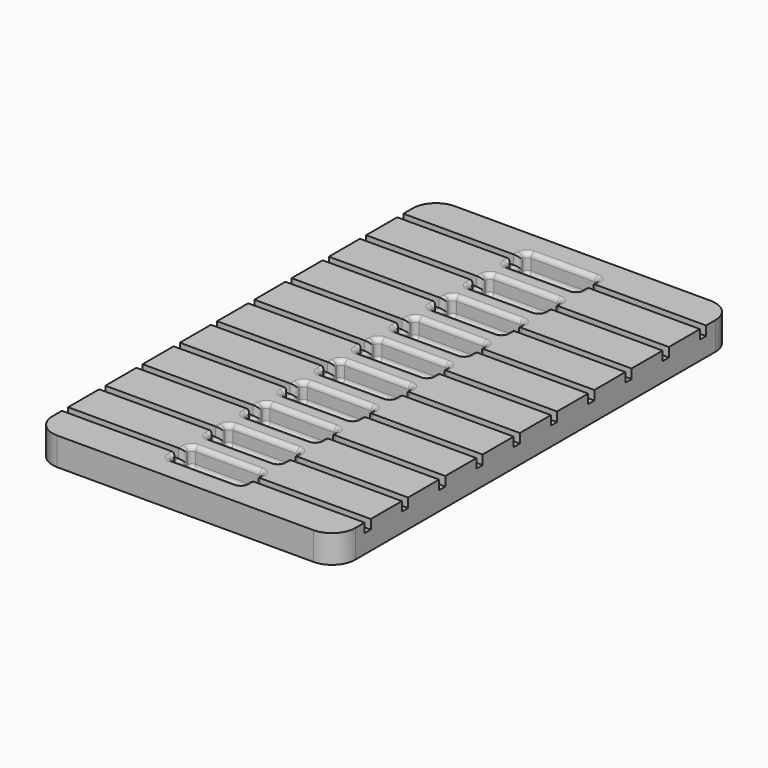
from build123d import *

# Parameters (mm, degrees)
F0_W     = 49.53
F0_H     = 81.28
F1_DEPTH = 4.572
F2_W     = 11.938
F2_H     = 4.572
F3_DEPTH = 3.302
F4_W     = 18.796
F4_H     = 1.27
F5_DEPTH = 1.524
F6_R     = 0.762
F7_R     = 3.81


with BuildPart() as f1:
    # F0 (on Top) → F1 (new body)
    with BuildSketch(Plane.XY):
        with Locations((24.765, 40.64)):
            Rectangle(F0_W, F0_H)
    extrude(amount=F1_DEPTH)

    # F2 (on face) → F3 (cut)
    with BuildSketch(Plane.XY.offset(4.572)):
        with Locations((24.765, 6.35)):
            Rectangle(F2_W, F2_H)
        with Locations((24.765, 13.97)):
            Rectangle(F2_W, F2_H)
        with Locations((24.765, 21.59)):
            Rectangle(F2_W, F2_H)
        with Locations((24.765, 29.21)):
            Rectangle(F2_W, F2_H)
        with Locations((24.765, 36.83)):
            Rectangle(F2_W, F2_H)
        with Locations((24.765, 44.45)):
            Rectangle(F2_W, F2_H)
        with Locations((24.765, 52.07)):
            Rectangle(F2_W, F2_H)
        with Locations((24.765, 59.69)):
            Rectangle(F2_W, F2_H)
        with Locations((24.765, 67.31)):
            Rectangle(F2_W, F2_H)
        with Locations((24.765, 74.93)):
            Rectangle(F2_W, F2_H)
    extrude(amount=-F3_DEPTH, mode=Mode.SUBTRACT)

    # F4 (on face) → F5 (cut)
    with BuildSketch(Plane.XY.offset(4.572)):
        with Locations((40.132, 6.35)):
            Rectangle(F4_W, F4_H)
        with Locations((9.398, 6.35)):
            Rectangle(F4_W, F4_H)
        with Locations((9.398, 13.97)):
            Rectangle(F4_W, F4_H)
        with Locations((40.132, 13.97)):
            Rectangle(F4_W, F4_H)
        with Locations((9.398, 21.59)):
            Rectangle(F4_W, F4_H)
        with Locations((40.132, 21.59)):
            Rectangle(F4_W, F4_H)
        with Locations((9.398, 29.21)):
            Rectangle(F4_W, F4_H)
        with Locations((40.132, 29.21)):
            Rectangle(F4_W, F4_H)
        with Locations((9.398, 36.83)):
            Rectangle(F4_W, F4_H)
        with Locations((40.132, 36.83)):
            Rectangle(F4_W, F4_H)
        with Locations((9.398, 44.45)):
            Rectangle(F4_W, F4_H)
        with Locations((40.132, 44.45)):
            Rectangle(F4_W, F4_H)
        with Locations((9.398, 52.07)):
            Rectangle(F4_W, F4_H)
        with Locations((40.132, 52.07)):
            Rectangle(F4_W, F4_H)
        with Locations((9.398, 59.69)):
            Rectangle(F4_W, F4_H)
        with Locations((40.132, 59.69)):
            Rectangle(F4_W, F4_H)
        with Locations((9.398, 67.31)):
            Rectangle(F4_W, F4_H)
        with Locations((40.132, 67.31)):
            Rectangle(F4_W, F4_H)
        with Locations((9.398, 74.93)):
            Rectangle(F4_W, F4_H)
        with Locations((40.132, 74.93)):
            Rectangle(F4_W, F4_H)
    extrude(amount=-F5_DEPTH, mode=Mode.SUBTRACT)

    # F6
    f6_edges = [f1.edges().sort_by_distance(p)[0] for p in [
        (18.796, 4.064, 2.921),
        (30.734, 4.064, 2.921),
        (24.765, 4.064, 4.572),
        (24.765, 4.064, 1.27),
        (18.796, 7.8105, 4.572),
        (18.796, 6.985, 3.81),
        (18.796, 6.35, 3.048),
        (18.796, 5.715, 3.81),
        (18.796, 4.8895, 4.572),
        (18.796, 6.35, 1.27),
        (18.796, 8.636, 2.921),
        (30.734, 4.8895, 4.572),
        (30.734, 5.715, 3.81),
        (30.734, 6.35, 3.048),
        (30.734, 6.985, 3.81),
        (30.734, 7.8105, 4.572),
        (30.734, 8.636, 2.921),
        (30.734, 6.35, 1.27),
        (24.765, 8.636, 4.572),
        (24.765, 8.636, 1.27),
        (18.796, 15.4305, 4.572),
        (18.796, 14.605, 3.81),
        (18.796, 13.97, 3.048),
        (18.796, 13.335, 3.81),
        (18.796, 12.5095, 4.572),
        (18.796, 11.684, 2.921),
        (18.796, 13.97, 1.27),
        (18.796, 16.256, 2.921),
        (18.796, 23.0505, 4.572),
        (18.796, 22.225, 3.81),
        (18.796, 21.59, 3.048),
        (18.796, 20.955, 3.81),
        (18.796, 20.1295, 4.572),
        (18.796, 19.304, 2.921),
        (18.796, 21.59, 1.27),
        (18.796, 23.876, 2.921),
        (18.796, 30.6705, 4.572),
        (18.796, 29.845, 3.81),
        (18.796, 29.21, 3.048),
        (18.796, 28.575, 3.81),
        (18.796, 27.7495, 4.572),
        (18.796, 26.924, 2.921),
        (18.796, 29.21, 1.27),
        (18.796, 31.496, 2.921),
        (18.796, 38.2905, 4.572),
        (18.796, 37.465, 3.81),
        (18.796, 36.83, 3.048),
        (18.796, 36.195, 3.81),
        (18.796, 35.3695, 4.572),
        (18.796, 34.544, 2.921),
        (18.796, 36.83, 1.27),
        (18.796, 39.116, 2.921),
        (18.796, 45.9105, 4.572),
        (18.796, 45.085, 3.81),
        (18.796, 44.45, 3.048),
        (18.796, 43.815, 3.81),
        (18.796, 42.9895, 4.572),
        (18.796, 42.164, 2.921),
        (18.796, 44.45, 1.27),
        (18.796, 46.736, 2.921),
        (18.796, 53.5305, 4.572),
        (18.796, 52.705, 3.81),
        (18.796, 52.07, 3.048),
        (18.796, 51.435, 3.81),
        (18.796, 50.6095, 4.572),
        (18.796, 49.784, 2.921),
        (18.796, 52.07, 1.27),
        (18.796, 54.356, 2.921),
        (18.796, 61.1505, 4.572),
        (18.796, 60.325, 3.81),
        (18.796, 59.69, 3.048),
        (18.796, 59.055, 3.81),
        (18.796, 58.2295, 4.572),
        (18.796, 57.404, 2.921),
        (18.796, 59.69, 1.27),
        (18.796, 61.976, 2.921),
        (18.796, 68.7705, 4.572),
        (18.796, 67.945, 3.81),
        (18.796, 67.31, 3.048),
        (18.796, 66.675, 3.81),
        (18.796, 65.8495, 4.572),
        (18.796, 65.024, 2.921),
        (18.796, 67.31, 1.27),
        (18.796, 69.596, 2.921),
        (18.796, 76.3905, 4.572),
        (18.796, 75.565, 3.81),
        (18.796, 74.93, 3.048),
        (18.796, 74.295, 3.81),
        (18.796, 73.4695, 4.572),
        (18.796, 72.644, 2.921),
        (18.796, 74.93, 1.27),
        (18.796, 77.216, 2.921),
        (30.734, 73.4695, 4.572),
        (30.734, 74.295, 3.81),
        (30.734, 74.93, 3.048),
        (30.734, 75.565, 3.81),
        (30.734, 76.3905, 4.572),
        (30.734, 77.216, 2.921),
        (30.734, 74.93, 1.27),
        (30.734, 72.644, 2.921),
        (30.734, 65.8495, 4.572),
        (30.734, 66.675, 3.81),
        (30.734, 67.31, 3.048),
        (30.734, 67.945, 3.81),
        (30.734, 68.7705, 4.572),
        (30.734, 69.596, 2.921),
        (30.734, 67.31, 1.27),
        (30.734, 65.024, 2.921),
        (30.734, 58.2295, 4.572),
        (30.734, 59.055, 3.81),
        (30.734, 59.69, 3.048),
        (30.734, 60.325, 3.81),
        (30.734, 61.1505, 4.572),
        (30.734, 61.976, 2.921),
        (30.734, 59.69, 1.27),
        (30.734, 57.404, 2.921),
        (30.734, 50.6095, 4.572),
        (30.734, 51.435, 3.81),
        (30.734, 52.07, 3.048),
        (30.734, 52.705, 3.81),
        (30.734, 53.5305, 4.572),
        (30.734, 54.356, 2.921),
        (30.734, 52.07, 1.27),
        (30.734, 49.784, 2.921),
        (30.734, 42.9895, 4.572),
        (30.734, 43.815, 3.81),
        (30.734, 44.45, 3.048),
        (30.734, 45.085, 3.81),
        (30.734, 45.9105, 4.572),
        (30.734, 46.736, 2.921),
        (30.734, 44.45, 1.27),
        (30.734, 42.164, 2.921),
        (30.734, 35.3695, 4.572),
        (30.734, 36.195, 3.81),
        (30.734, 36.83, 3.048),
        (30.734, 37.465, 3.81),
        (30.734, 38.2905, 4.572),
        (30.734, 39.116, 2.921),
        (30.734, 36.83, 1.27),
        (30.734, 34.544, 2.921),
        (30.734, 27.7495, 4.572),
        (30.734, 28.575, 3.81),
        (30.734, 29.21, 3.048),
        (30.734, 29.845, 3.81),
        (30.734, 30.6705, 4.572),
        (30.734, 31.496, 2.921),
        (30.734, 29.21, 1.27),
        (30.734, 26.924, 2.921),
        (30.734, 20.1295, 4.572),
        (30.734, 20.955, 3.81),
        (30.734, 21.59, 3.048),
        (30.734, 22.225, 3.81),
        (30.734, 23.0505, 4.572),
        (30.734, 23.876, 2.921),
        (30.734, 21.59, 1.27),
        (30.734, 19.304, 2.921),
        (30.734, 12.5095, 4.572),
        (30.734, 13.335, 3.81),
        (30.734, 13.97, 3.048),
        (30.734, 14.605, 3.81),
        (30.734, 15.4305, 4.572),
        (30.734, 16.256, 2.921),
        (30.734, 13.97, 1.27),
        (30.734, 11.684, 2.921),
        (24.765, 11.684, 4.572),
        (24.765, 11.684, 1.27),
        (24.765, 16.256, 4.572),
        (24.765, 16.256, 1.27),
        (24.765, 23.876, 1.27),
        (24.765, 19.304, 1.27),
        (24.765, 31.496, 1.27),
        (24.765, 26.924, 1.27),
        (24.765, 39.116, 1.27),
        (24.765, 34.544, 1.27),
        (24.765, 46.736, 1.27),
        (24.765, 42.164, 1.27),
        (24.765, 54.356, 1.27),
        (24.765, 49.784, 1.27),
        (24.765, 61.976, 1.27),
        (24.765, 57.404, 1.27),
        (24.765, 69.596, 1.27),
        (24.765, 65.024, 1.27),
        (24.765, 77.216, 1.27),
        (24.765, 72.644, 1.27),
        (24.765, 19.304, 4.572),
        (24.765, 26.924, 4.572),
        (24.765, 23.876, 4.572),
        (24.765, 34.544, 4.572),
        (24.765, 31.496, 4.572),
        (24.765, 42.164, 4.572),
        (24.765, 39.116, 4.572),
        (24.765, 49.784, 4.572),
        (24.765, 46.736, 4.572),
        (24.765, 57.404, 4.572),
        (24.765, 54.356, 4.572),
        (24.765, 65.024, 4.572),
        (24.765, 61.976, 4.572),
        (24.765, 72.644, 4.572),
        (24.765, 69.596, 4.572),
        (24.765, 77.216, 4.572),
    ]]
    fillet(f6_edges, radius=F6_R)

    # F7
    f7_edges = [f1.edges().sort_by_distance(p)[0] for p in [
        (49.53, 0, 2.286),
        (0, 0, 2.286),
        (0, 81.28, 2.286),
        (49.53, 81.28, 2.286),
    ]]
    fillet(f7_edges, radius=F7_R)


solid = f1.part
